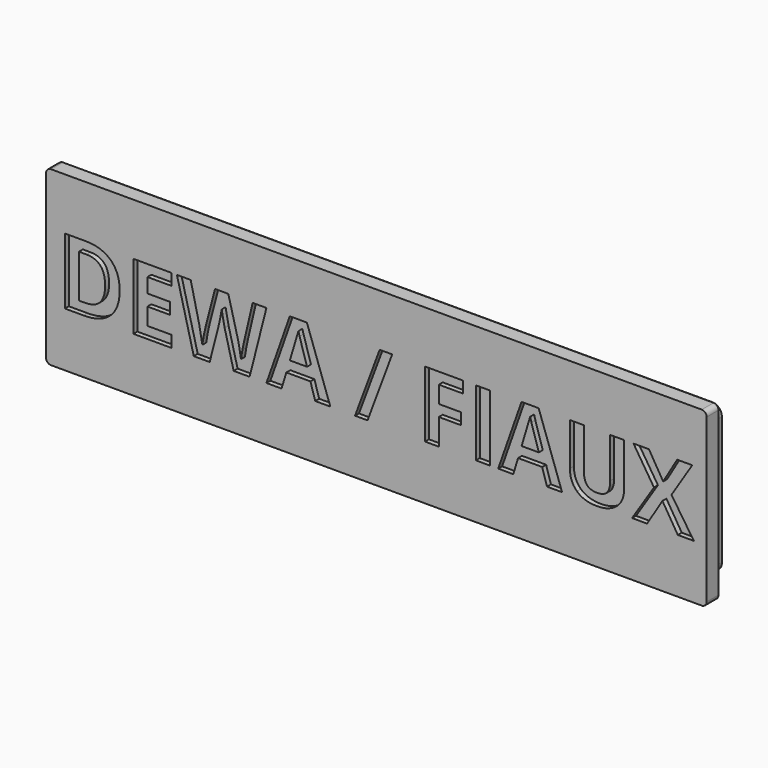
from build123d import *

# Parameters (mm, degrees)
F0_W         = 2.843732235
F0_H         = 13.4086817149
F0_TEXT_SIZE = 18.7821324087
F1_DEPTH     = 2
F2_DEPTH     = 1
F3_R         = 1.35
F4_DEPTH     = 3.8


# Not quite as in the source:
# - Text() gives the source's letters only with a copy of the font that has no kerning and outlines rounded to 1/6400 em; it was checked with that copy


with BuildPart() as f1:
    # F0 (on Front) → F1 (new body)
    with BuildSketch(Plane.XZ):
        with BuildLine():
            ThreePointArc((0, 1), (0.2928932188, 0.2928932188), (1, 0))
            Line((1, 0), (133, 0))
            ThreePointArc((133, 0), (133.7071067812, 0.2928932188), (134, 1))
            Line((134, 1), (134, 34))
            ThreePointArc((134, 34), (133.7071067812, 34.7071067812), (133, 35))
            Line((133, 35), (1, 35))
            ThreePointArc((1, 35), (0.2928932188, 34.7071067812), (0, 34))
            Line((0, 34), (0, 1))
        make_face()
        with BuildLine():
            add(Edge.make_bspline(
                [(13.111640333, 22.7105586208), (14.9282247019, 20.9776134353), (14.9282247019, 17.8668227551)],
                knots=[0, 0, 0, 1, 1, 1], degree=2))
            add(Edge.make_bspline(
                [(14.9282247019, 17.8668227551), (14.9282247019, 14.5564719181), (13.0426746905, 12.7956470048)],
                knots=[0, 0, 0, 1, 1, 1], degree=2))
            add(Edge.make_bspline(
                [(13.0426746905, 12.7956470048), (11.1571246792, 11.0348220915), (7.6002583543, 11.0348220915)],
                knots=[0, 0, 0, 1, 1, 1], degree=2))
            Line((7.6002583543, 11.0348220915), (3.8027459579, 11.0348220915))
            Line((3.8027459579, 11.0348220915), (3.8027459579, 24.4435038063))
            Line((3.8027459579, 24.4435038063), (8.0111175008, 24.4435038063))
            add(Edge.make_bspline(
                [(8.0111175008, 24.4435038063), (11.2950559641, 24.4435038063), (13.111640333, 22.7105586208)],
                knots=[0, 0, 0, 1, 1, 1], degree=2))
        make_face(mode=Mode.SUBTRACT)
        Polygon((25.4286106016, 13.3825886425), (25.4286106016, 11.0348220915), (17.7073933567, 11.0348220915), (17.7073933567, 24.4435038063), (25.4286106016, 24.4435038063), (25.4286106016, 22.1133455044), (20.5511255917, 22.1133455044), (20.5511255917, 19.169833191), (25.0911191599, 19.169833191), (25.0911191599, 16.839674889), (20.5511255917, 16.839674889), (20.5511255917, 13.3825886425), align=None, mode=Mode.SUBTRACT)
        with BuildLine():
            Line((44.6979045697, 24.4435038063), (41.284838946, 11.0348220915))
            Line((41.284838946, 11.0348220915), (38.0478558137, 11.0348220915))
            Line((38.0478558137, 11.0348220915), (36.2312714448, 18.0781217447))
            add(Edge.make_bspline(
                [(36.2312714448, 18.0781217447), (36.1314913664, 18.4537643929), (35.8879105867, 19.6320497307)],
                knots=[0, 0, 0, 1, 1, 1], degree=2))
            add(Edge.make_bspline(
                [(35.8879105867, 19.6320497307), (35.644329807, 20.8103350685), (35.6091133088, 21.2153247986)],
                knots=[0, 0, 0, 1, 1, 1], degree=2))
            add(Edge.make_bspline(
                [(35.6091133088, 21.2153247986), (35.5533538532, 20.7193591147), (35.333250739, 19.6232456062)],
                knots=[0, 0, 0, 1, 1, 1], degree=2))
            add(Edge.make_bspline(
                [(35.333250739, 19.6232456062), (35.1131476248, 18.5271320976), (34.9928245891, 18.0605134956)],
                knots=[0, 0, 0, 1, 1, 1], degree=2))
            Line((34.9928245891, 18.0605134956), (33.187979053, 11.0348220915))
            Line((33.187979053, 11.0348220915), (29.9598000452, 11.0348220915))
            Line((29.9598000452, 11.0348220915), (26.537930297, 24.4435038063))
            Line((26.537930297, 24.4435038063), (29.334707201, 24.4435038063))
            Line((29.334707201, 24.4435038063), (31.0515114915, 17.1243415833))
            add(Edge.make_bspline(
                [(31.0515114915, 17.1243415833), (31.5005218444, 15.0964582248), (31.7000820012, 13.6114958813)],
                knots=[0, 0, 0, 1, 1, 1], degree=2))
            add(Edge.make_bspline(
                [(31.7000820012, 13.6114958813), (31.7558414568, 14.1338739389), (31.9539342595, 15.2299874474)],
                knots=[0, 0, 0, 1, 1, 1], degree=2))
            add(Edge.make_bspline(
                [(31.9539342595, 15.2299874474), (32.1520270623, 16.326100956), (32.3251748454, 16.9306508429)],
                knots=[0, 0, 0, 1, 1, 1], degree=2))
            Line((32.3251748454, 16.9306508429), (34.2796904992, 24.4435038063))
            Line((34.2796904992, 24.4435038063), (36.964948492, 24.4435038063))
            Line((36.964948492, 24.4435038063), (38.9194641458, 16.9306508429))
            add(Edge.make_bspline(
                [(38.9194641458, 16.9306508429), (39.0485913061, 16.4288157426), (39.2408146925, 15.3913963978)],
                knots=[0, 0, 0, 1, 1, 1], degree=2))
            add(Edge.make_bspline(
                [(39.2408146925, 15.3913963978), (39.4330380788, 14.3539770531), (39.5328181573, 13.6114958813)],
                knots=[0, 0, 0, 1, 1, 1], degree=2))
            add(Edge.make_bspline(
                [(39.5328181573, 13.6114958813), (39.6237941111, 14.3275646794), (39.8262889762, 15.3957984601)],
                knots=[0, 0, 0, 1, 1, 1], degree=2))
            add(Edge.make_bspline(
                [(39.8262889762, 15.3957984601), (40.0287838412, 16.4640322408), (40.1931274998, 17.1243415833)],
                knots=[0, 0, 0, 1, 1, 1], degree=2))
            Line((40.1931274998, 17.1243415833), (41.8981929575, 24.4435038063))
            Line((41.8981929575, 24.4435038063), (44.6979045697, 24.4435038063))
        make_face(mode=Mode.SUBTRACT)
        Polygon((57.6575759316, 11.0348220915), (54.5937405825, 11.0348220915), (53.622352172, 14.2277846009), (48.7331283293, 14.2277846009), (47.7617399188, 11.0348220915), (44.6979045697, 11.0348220915), (49.4315888783, 24.4992632619), (52.9062833739, 24.4992632619), align=None, mode=Mode.SUBTRACT)
        Polygon((67.6649308556, 24.4435038063), (70.2063881472, 24.4435038063), (65.2056453934, 11.0348220915), (62.66712281, 11.0348220915), align=None, mode=Mode.SUBTRACT)
        Polygon((79.6620179317, 16.3349050805), (79.6620179317, 11.0348220915), (76.8652410277, 11.0348220915), (76.8652410277, 24.4435038063), (84.5512417743, 24.4435038063), (84.5512417743, 22.1133455044), (79.6620179317, 22.1133455044), (79.6620179317, 18.6562592579), (84.2108156244, 18.6562592579), (84.2108156244, 16.3349050805), align=None, mode=Mode.SUBTRACT)
        with Locations((88.5967370127, 17.7391629489)):
            Rectangle(F0_W, F0_H, mode=Mode.SUBTRACT)
        Polygon((104.6657317008, 11.0348220915), (101.6018963516, 11.0348220915), (100.6305079411, 14.2277846009), (95.7412840984, 14.2277846009), (94.7698956879, 11.0348220915), (91.7060603388, 11.0348220915), (96.4397446474, 24.4992632619), (99.914439143, 24.4992632619), align=None, mode=Mode.SUBTRACT)
        with BuildLine():
            Line((114.4324405533, 24.4435038063), (117.2673686637, 24.4435038063))
            Line((117.2673686637, 24.4435038063), (117.2673686637, 15.7685064001))
            add(Edge.make_bspline(
                [(117.2673686637, 15.7685064001), (117.2673686637, 14.2806093483), (116.6026572589, 13.1624855284)],
                knots=[0, 0, 0, 1, 1, 1], degree=2))
            add(Edge.make_bspline(
                [(116.6026572589, 13.1624855284), (115.9379458542, 12.0443617084), (114.6804233952, 11.447148592)],
                knots=[0, 0, 0, 1, 1, 1], degree=2))
            add(Edge.make_bspline(
                [(114.6804233952, 11.447148592), (113.4229009363, 10.8499354756), (111.709031354, 10.8499354756)],
                knots=[0, 0, 0, 1, 1, 1], degree=2))
            add(Edge.make_bspline(
                [(111.709031354, 10.8499354756), (109.1235534396, 10.8499354756), (107.6928831976, 12.1764235769)],
                knots=[0, 0, 0, 1, 1, 1], degree=2))
            add(Edge.make_bspline(
                [(107.6928831976, 12.1764235769), (106.2622129555, 13.5029116783), (106.2622129555, 15.8037228984)],
                knots=[0, 0, 0, 1, 1, 1], degree=2))
            Line((106.2622129555, 15.8037228984), (106.2622129555, 24.4435038063))
            Line((106.2622129555, 24.4435038063), (109.0942063577, 24.4435038063))
            Line((109.0942063577, 24.4435038063), (109.0942063577, 16.2351250021))
            add(Edge.make_bspline(
                [(109.0942063577, 16.2351250021), (109.0942063577, 14.6855990784), (109.7178318479, 13.9607261558)],
                knots=[0, 0, 0, 1, 1, 1], degree=2))
            add(Edge.make_bspline(
                [(109.7178318479, 13.9607261558), (110.341457338, 13.2358532331), (111.7823990587, 13.2358532331)],
                knots=[0, 0, 0, 1, 1, 1], degree=2))
            add(Edge.make_bspline(
                [(111.7823990587, 13.2358532331), (113.1763854484, 13.2358532331), (113.8044130009, 13.965128218)],
                knots=[0, 0, 0, 1, 1, 1], degree=2))
            add(Edge.make_bspline(
                [(113.8044130009, 13.965128218), (114.4324405533, 14.694403203), (114.4324405533, 16.2527332512)],
                knots=[0, 0, 0, 1, 1, 1], degree=2))
            Line((114.4324405533, 16.2527332512), (114.4324405533, 24.4435038063))
        make_face(mode=Mode.SUBTRACT)
        Polygon((126.8609297331, 17.7934550504), (131.3921191767, 11.0348220915), (128.1463319198, 11.0348220915), (125.026737115, 16.1059978418), (121.9100770185, 11.0348220915), (118.8638499184, 11.0348220915), (123.3128675328, 17.9489945844), (119.1485166128, 24.4435038063), (122.2857196667, 24.4435038063), (125.1734725245, 19.6188435439), (128.0084006349, 24.4435038063), (131.0693012759, 24.4435038063), align=None, mode=Mode.SUBTRACT)
        with BuildLine():
            add(Edge.make_bspline(
                [(7.8643820913, 13.3825886425), (11.9729735557, 13.3825886425), (11.9729735557, 17.7934550504)],
                knots=[0, 0, 0, 1, 1, 1], degree=2))
            add(Edge.make_bspline(
                [(11.9729735557, 17.7934550504), (11.9729735557, 22.1133455044), (8.1578529102, 22.1133455044)],
                knots=[0, 0, 0, 1, 1, 1], degree=2))
            Line((8.1578529102, 22.1133455044), (6.6464781929, 22.1133455044))
            Line((6.6464781929, 22.1133455044), (6.6464781929, 13.3825886425))
            Line((6.6464781929, 13.3825886425), (7.8643820913, 13.3825886425))
        make_face()
        with Locations((2.1152887493, 11.0348220915)):
            Text('DEWA / FIAUX', F0_TEXT_SIZE, font='Open Sans', font_style=FontStyle.BOLD, text_align=(TextAlign.LEFT, TextAlign.BOTTOM))
        with BuildLine():
            Line((49.4491971274, 16.6107676503), (52.9414998722, 16.6107676503))
            add(Edge.make_bspline(
                [(52.9414998722, 16.6107676503), (51.5944688135, 20.9482663534), (51.4242557385, 21.5175997421)],
                knots=[0, 0, 0, 1, 1, 1], degree=2))
            add(Edge.make_bspline(
                [(51.4242557385, 21.5175997421), (51.2540426636, 22.0869331307), (51.1806749588, 22.4156204478)],
                knots=[0, 0, 0, 1, 1, 1], degree=2))
            add(Edge.make_bspline(
                [(51.1806749588, 22.4156204478), (50.8784000154, 21.2417371723), (49.4491971274, 16.6107676503)],
                knots=[0, 0, 0, 1, 1, 1], degree=2))
        make_face()
        with BuildLine():
            Line((96.4573528965, 16.6107676503), (99.9496556413, 16.6107676503))
            add(Edge.make_bspline(
                [(99.9496556413, 16.6107676503), (98.6026245826, 20.9482663534), (98.4324115076, 21.5175997421)],
                knots=[0, 0, 0, 1, 1, 1], degree=2))
            add(Edge.make_bspline(
                [(98.4324115076, 21.5175997421), (98.2621984327, 22.0869331307), (98.188830728, 22.4156204478)],
                knots=[0, 0, 0, 1, 1, 1], degree=2))
            add(Edge.make_bspline(
                [(98.188830728, 22.4156204478), (97.8865557845, 21.2417371723), (96.4573528965, 16.6107676503)],
                knots=[0, 0, 0, 1, 1, 1], degree=2))
        make_face()
    extrude(amount=-F1_DEPTH)

    # F0 (on Front) → F2 (join)
    with BuildSketch(Plane.XZ):
        with BuildLine():
            ThreePointArc((0, 1), (0.2928932188, 0.2928932188), (1, 0))
            Line((1, 0), (133, 0))
            ThreePointArc((133, 0), (133.7071067812, 0.2928932188), (134, 1))
            Line((134, 1), (134, 34))
            ThreePointArc((134, 34), (133.7071067812, 34.7071067812), (133, 35))
            Line((133, 35), (1, 35))
            ThreePointArc((1, 35), (0.2928932188, 34.7071067812), (0, 34))
            Line((0, 34), (0, 1))
        make_face()
        with BuildLine():
            add(Edge.make_bspline(
                [(13.111640333, 22.7105586208), (14.9282247019, 20.9776134353), (14.9282247019, 17.8668227551)],
                knots=[0, 0, 0, 1, 1, 1], degree=2))
            add(Edge.make_bspline(
                [(14.9282247019, 17.8668227551), (14.9282247019, 14.5564719181), (13.0426746905, 12.7956470048)],
                knots=[0, 0, 0, 1, 1, 1], degree=2))
            add(Edge.make_bspline(
                [(13.0426746905, 12.7956470048), (11.1571246792, 11.0348220915), (7.6002583543, 11.0348220915)],
                knots=[0, 0, 0, 1, 1, 1], degree=2))
            Line((7.6002583543, 11.0348220915), (3.8027459579, 11.0348220915))
            Line((3.8027459579, 11.0348220915), (3.8027459579, 24.4435038063))
            Line((3.8027459579, 24.4435038063), (8.0111175008, 24.4435038063))
            add(Edge.make_bspline(
                [(8.0111175008, 24.4435038063), (11.2950559641, 24.4435038063), (13.111640333, 22.7105586208)],
                knots=[0, 0, 0, 1, 1, 1], degree=2))
        make_face(mode=Mode.SUBTRACT)
        Polygon((25.4286106016, 13.3825886425), (25.4286106016, 11.0348220915), (17.7073933567, 11.0348220915), (17.7073933567, 24.4435038063), (25.4286106016, 24.4435038063), (25.4286106016, 22.1133455044), (20.5511255917, 22.1133455044), (20.5511255917, 19.169833191), (25.0911191599, 19.169833191), (25.0911191599, 16.839674889), (20.5511255917, 16.839674889), (20.5511255917, 13.3825886425), align=None, mode=Mode.SUBTRACT)
        with BuildLine():
            Line((44.6979045697, 24.4435038063), (41.284838946, 11.0348220915))
            Line((41.284838946, 11.0348220915), (38.0478558137, 11.0348220915))
            Line((38.0478558137, 11.0348220915), (36.2312714448, 18.0781217447))
            add(Edge.make_bspline(
                [(36.2312714448, 18.0781217447), (36.1314913664, 18.4537643929), (35.8879105867, 19.6320497307)],
                knots=[0, 0, 0, 1, 1, 1], degree=2))
            add(Edge.make_bspline(
                [(35.8879105867, 19.6320497307), (35.644329807, 20.8103350685), (35.6091133088, 21.2153247986)],
                knots=[0, 0, 0, 1, 1, 1], degree=2))
            add(Edge.make_bspline(
                [(35.6091133088, 21.2153247986), (35.5533538532, 20.7193591147), (35.333250739, 19.6232456062)],
                knots=[0, 0, 0, 1, 1, 1], degree=2))
            add(Edge.make_bspline(
                [(35.333250739, 19.6232456062), (35.1131476248, 18.5271320976), (34.9928245891, 18.0605134956)],
                knots=[0, 0, 0, 1, 1, 1], degree=2))
            Line((34.9928245891, 18.0605134956), (33.187979053, 11.0348220915))
            Line((33.187979053, 11.0348220915), (29.9598000452, 11.0348220915))
            Line((29.9598000452, 11.0348220915), (26.537930297, 24.4435038063))
            Line((26.537930297, 24.4435038063), (29.334707201, 24.4435038063))
            Line((29.334707201, 24.4435038063), (31.0515114915, 17.1243415833))
            add(Edge.make_bspline(
                [(31.0515114915, 17.1243415833), (31.5005218444, 15.0964582248), (31.7000820012, 13.6114958813)],
                knots=[0, 0, 0, 1, 1, 1], degree=2))
            add(Edge.make_bspline(
                [(31.7000820012, 13.6114958813), (31.7558414568, 14.1338739389), (31.9539342595, 15.2299874474)],
                knots=[0, 0, 0, 1, 1, 1], degree=2))
            add(Edge.make_bspline(
                [(31.9539342595, 15.2299874474), (32.1520270623, 16.326100956), (32.3251748454, 16.9306508429)],
                knots=[0, 0, 0, 1, 1, 1], degree=2))
            Line((32.3251748454, 16.9306508429), (34.2796904992, 24.4435038063))
            Line((34.2796904992, 24.4435038063), (36.964948492, 24.4435038063))
            Line((36.964948492, 24.4435038063), (38.9194641458, 16.9306508429))
            add(Edge.make_bspline(
                [(38.9194641458, 16.9306508429), (39.0485913061, 16.4288157426), (39.2408146925, 15.3913963978)],
                knots=[0, 0, 0, 1, 1, 1], degree=2))
            add(Edge.make_bspline(
                [(39.2408146925, 15.3913963978), (39.4330380788, 14.3539770531), (39.5328181573, 13.6114958813)],
                knots=[0, 0, 0, 1, 1, 1], degree=2))
            add(Edge.make_bspline(
                [(39.5328181573, 13.6114958813), (39.6237941111, 14.3275646794), (39.8262889762, 15.3957984601)],
                knots=[0, 0, 0, 1, 1, 1], degree=2))
            add(Edge.make_bspline(
                [(39.8262889762, 15.3957984601), (40.0287838412, 16.4640322408), (40.1931274998, 17.1243415833)],
                knots=[0, 0, 0, 1, 1, 1], degree=2))
            Line((40.1931274998, 17.1243415833), (41.8981929575, 24.4435038063))
            Line((41.8981929575, 24.4435038063), (44.6979045697, 24.4435038063))
        make_face(mode=Mode.SUBTRACT)
        Polygon((57.6575759316, 11.0348220915), (54.5937405825, 11.0348220915), (53.622352172, 14.2277846009), (48.7331283293, 14.2277846009), (47.7617399188, 11.0348220915), (44.6979045697, 11.0348220915), (49.4315888783, 24.4992632619), (52.9062833739, 24.4992632619), align=None, mode=Mode.SUBTRACT)
        Polygon((67.6649308556, 24.4435038063), (70.2063881472, 24.4435038063), (65.2056453934, 11.0348220915), (62.66712281, 11.0348220915), align=None, mode=Mode.SUBTRACT)
        Polygon((79.6620179317, 16.3349050805), (79.6620179317, 11.0348220915), (76.8652410277, 11.0348220915), (76.8652410277, 24.4435038063), (84.5512417743, 24.4435038063), (84.5512417743, 22.1133455044), (79.6620179317, 22.1133455044), (79.6620179317, 18.6562592579), (84.2108156244, 18.6562592579), (84.2108156244, 16.3349050805), align=None, mode=Mode.SUBTRACT)
        with Locations((88.5967370127, 17.7391629489)):
            Rectangle(F0_W, F0_H, mode=Mode.SUBTRACT)
        Polygon((104.6657317008, 11.0348220915), (101.6018963516, 11.0348220915), (100.6305079411, 14.2277846009), (95.7412840984, 14.2277846009), (94.7698956879, 11.0348220915), (91.7060603388, 11.0348220915), (96.4397446474, 24.4992632619), (99.914439143, 24.4992632619), align=None, mode=Mode.SUBTRACT)
        with BuildLine():
            Line((114.4324405533, 24.4435038063), (117.2673686637, 24.4435038063))
            Line((117.2673686637, 24.4435038063), (117.2673686637, 15.7685064001))
            add(Edge.make_bspline(
                [(117.2673686637, 15.7685064001), (117.2673686637, 14.2806093483), (116.6026572589, 13.1624855284)],
                knots=[0, 0, 0, 1, 1, 1], degree=2))
            add(Edge.make_bspline(
                [(116.6026572589, 13.1624855284), (115.9379458542, 12.0443617084), (114.6804233952, 11.447148592)],
                knots=[0, 0, 0, 1, 1, 1], degree=2))
            add(Edge.make_bspline(
                [(114.6804233952, 11.447148592), (113.4229009363, 10.8499354756), (111.709031354, 10.8499354756)],
                knots=[0, 0, 0, 1, 1, 1], degree=2))
            add(Edge.make_bspline(
                [(111.709031354, 10.8499354756), (109.1235534396, 10.8499354756), (107.6928831976, 12.1764235769)],
                knots=[0, 0, 0, 1, 1, 1], degree=2))
            add(Edge.make_bspline(
                [(107.6928831976, 12.1764235769), (106.2622129555, 13.5029116783), (106.2622129555, 15.8037228984)],
                knots=[0, 0, 0, 1, 1, 1], degree=2))
            Line((106.2622129555, 15.8037228984), (106.2622129555, 24.4435038063))
            Line((106.2622129555, 24.4435038063), (109.0942063577, 24.4435038063))
            Line((109.0942063577, 24.4435038063), (109.0942063577, 16.2351250021))
            add(Edge.make_bspline(
                [(109.0942063577, 16.2351250021), (109.0942063577, 14.6855990784), (109.7178318479, 13.9607261558)],
                knots=[0, 0, 0, 1, 1, 1], degree=2))
            add(Edge.make_bspline(
                [(109.7178318479, 13.9607261558), (110.341457338, 13.2358532331), (111.7823990587, 13.2358532331)],
                knots=[0, 0, 0, 1, 1, 1], degree=2))
            add(Edge.make_bspline(
                [(111.7823990587, 13.2358532331), (113.1763854484, 13.2358532331), (113.8044130009, 13.965128218)],
                knots=[0, 0, 0, 1, 1, 1], degree=2))
            add(Edge.make_bspline(
                [(113.8044130009, 13.965128218), (114.4324405533, 14.694403203), (114.4324405533, 16.2527332512)],
                knots=[0, 0, 0, 1, 1, 1], degree=2))
            Line((114.4324405533, 16.2527332512), (114.4324405533, 24.4435038063))
        make_face(mode=Mode.SUBTRACT)
        Polygon((126.8609297331, 17.7934550504), (131.3921191767, 11.0348220915), (128.1463319198, 11.0348220915), (125.026737115, 16.1059978418), (121.9100770185, 11.0348220915), (118.8638499184, 11.0348220915), (123.3128675328, 17.9489945844), (119.1485166128, 24.4435038063), (122.2857196667, 24.4435038063), (125.1734725245, 19.6188435439), (128.0084006349, 24.4435038063), (131.0693012759, 24.4435038063), align=None, mode=Mode.SUBTRACT)
        with BuildLine():
            add(Edge.make_bspline(
                [(7.8643820913, 13.3825886425), (11.9729735557, 13.3825886425), (11.9729735557, 17.7934550504)],
                knots=[0, 0, 0, 1, 1, 1], degree=2))
            add(Edge.make_bspline(
                [(11.9729735557, 17.7934550504), (11.9729735557, 22.1133455044), (8.1578529102, 22.1133455044)],
                knots=[0, 0, 0, 1, 1, 1], degree=2))
            Line((8.1578529102, 22.1133455044), (6.6464781929, 22.1133455044))
            Line((6.6464781929, 22.1133455044), (6.6464781929, 13.3825886425))
            Line((6.6464781929, 13.3825886425), (7.8643820913, 13.3825886425))
        make_face()
        with BuildLine():
            Line((49.4491971274, 16.6107676503), (52.9414998722, 16.6107676503))
            add(Edge.make_bspline(
                [(52.9414998722, 16.6107676503), (51.5944688135, 20.9482663534), (51.4242557385, 21.5175997421)],
                knots=[0, 0, 0, 1, 1, 1], degree=2))
            add(Edge.make_bspline(
                [(51.4242557385, 21.5175997421), (51.2540426636, 22.0869331307), (51.1806749588, 22.4156204478)],
                knots=[0, 0, 0, 1, 1, 1], degree=2))
            add(Edge.make_bspline(
                [(51.1806749588, 22.4156204478), (50.8784000154, 21.2417371723), (49.4491971274, 16.6107676503)],
                knots=[0, 0, 0, 1, 1, 1], degree=2))
        make_face()
        with BuildLine():
            Line((96.4573528965, 16.6107676503), (99.9496556413, 16.6107676503))
            add(Edge.make_bspline(
                [(99.9496556413, 16.6107676503), (98.6026245826, 20.9482663534), (98.4324115076, 21.5175997421)],
                knots=[0, 0, 0, 1, 1, 1], degree=2))
            add(Edge.make_bspline(
                [(98.4324115076, 21.5175997421), (98.2621984327, 22.0869331307), (98.188830728, 22.4156204478)],
                knots=[0, 0, 0, 1, 1, 1], degree=2))
            add(Edge.make_bspline(
                [(98.188830728, 22.4156204478), (97.8865557845, 21.2417371723), (96.4573528965, 16.6107676503)],
                knots=[0, 0, 0, 1, 1, 1], degree=2))
        make_face()
    extrude(amount=F2_DEPTH)

    # F3 (on face) → F4 (join)
    with BuildSketch(Plane(origin=(0, 2, 0), x_dir=(-1, 0, 0), z_dir=(0, 1, 0))):
        with BuildLine():
            Line((-4.35, 32.5), (-129.65, 32.5))
            ThreePointArc((-129.65, 32.5), (-131.0642135624, 31.9142135624), (-131.65, 30.5))
            Line((-131.65, 30.5), (-131.65, 20.5))
            Line((-131.65, 20.5), (-131.65, 14.5))
            Line((-131.65, 14.5), (-131.65, 4.5))
            ThreePointArc((-131.65, 4.5), (-131.0642135624, 3.0857864376), (-129.65, 2.5))
            Line((-129.65, 2.5), (-4.35, 2.5))
            ThreePointArc((-4.35, 2.5), (-2.9357864376, 3.0857864376), (-2.35, 4.5))
            Line((-2.35, 4.5), (-2.35, 30.5))
            ThreePointArc((-2.35, 30.5), (-2.9357864376, 31.9142135624), (-4.35, 32.5))
        make_face()
        with Locations((-129.15, 17.5)):
            Circle(F3_R, mode=Mode.SUBTRACT)
        with BuildLine():
            ThreePointArc((-129.15, 28), (-128.5642135624, 29.4142135624), (-127.15, 30))
            Line((-127.15, 30), (-67, 30))
            Line((-67, 30), (-6.85, 30))
            ThreePointArc((-6.85, 30), (-5.4357864376, 29.4142135624), (-4.85, 28))
            Line((-4.85, 28), (-4.85, 20.5))
            Line((-4.85, 20.5), (-7.85, 20.5))
            Line((-7.85, 20.5), (-7.85, 14.5))
            Line((-7.85, 14.5), (-4.85, 14.5))
            Line((-4.85, 14.5), (-4.85, 7))
            ThreePointArc((-4.85, 7), (-5.4357864376, 5.5857864376), (-6.85, 5))
            Line((-6.85, 5), (-67, 5))
            Line((-67, 5), (-127.15, 5))
            ThreePointArc((-127.15, 5), (-128.5642135624, 5.5857864376), (-129.15, 7))
            Line((-129.15, 7), (-129.15, 14.5))
            Line((-129.15, 14.5), (-126.15, 14.5))
            Line((-126.15, 14.5), (-126.15, 20.5))
            Line((-126.15, 20.5), (-129.15, 20.5))
            Line((-129.15, 20.5), (-129.15, 28))
        make_face(mode=Mode.SUBTRACT)
        with Locations((-4.85, 17.5)):
            Circle(F3_R, mode=Mode.SUBTRACT)
    extrude(amount=F4_DEPTH)


solid = f1.part
